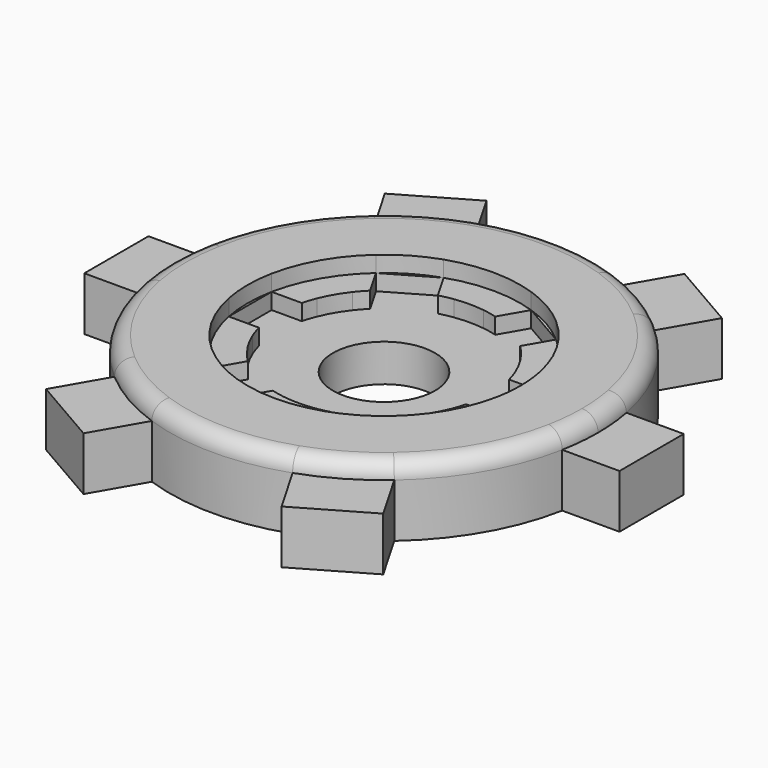
from build123d import *

# Parameters (mm, degrees)
F2_DEPTH = 2.54
F3_R     = 7.6884407039
F3_R_2   = 2.4226171542
F4_DEPTH = 1.778
F6_DEPTH = 0.762
F7_R     = 0.76199


# Not quite as in the source:
# - a fillet or chamfer is up to 0.001 mm smaller than in the source, because OpenCascade refuses the exact size


with BuildPart() as f2:
    # F1 (on Top) → F2 (new body)
    with BuildSketch(Plane.XY):
        with BuildLine():
            ThreePointArc((9.9798083649, -1.905), (10.1148517781, -0.9567515385), (10.16, 0))
            ThreePointArc((10.16, 0), (10.1148517781, 0.9567515385), (9.9798083649, 1.905))
            Line((9.9798083649, 1.905), (4.7092860393, 1.905))
            ThreePointArc((4.7092860393, 1.905), (4.8244462237, 1.5909489729), (4.9186888497, 1.27))
            Line((4.9186888497, 1.27), (6.35, 1.27))
            Line((6.35, 1.27), (6.35, -1.27))
            Line((6.35, -1.27), (4.9186888497, -1.27))
            ThreePointArc((4.9186888497, -1.27), (4.8244462237, -1.5909489729), (4.7092860393, -1.905))
            Line((4.7092860393, -1.905), (9.9798083649, -1.905))
        make_face()
        with BuildLine():
            ThreePointArc((9.9798083649, 1.905), (10.1148517781, 0.9567515385), (10.16, 0))
            ThreePointArc((10.16, 0), (10.1148517781, -0.9567515385), (9.9798083649, -1.905))
            Line((9.9798083649, -1.905), (12.7, -1.905))
            Line((12.7, -1.905), (12.7, 1.905))
            Line((12.7, 1.905), (9.9798083649, 1.905))
        make_face()
        with BuildLine():
            Line((4.7092860393, 1.905), (9.9798083649, 1.905))
            ThreePointArc((9.9798083649, 1.905), (8.7988181024, 5.08), (6.6396825767, 7.6902675689))
            Line((6.6396825767, 7.6902675689), (4.0044214139, 3.1258613437))
            ThreePointArc((4.0044214139, 3.1258613437), (4.3994090512, 2.54), (4.7092860393, 1.905))
        make_face()
        with BuildLine():
            ThreePointArc((6.6396825767, -7.6902675689), (8.7988181024, -5.08), (9.9798083649, -1.905))
            Line((9.9798083649, -1.905), (4.7092860393, -1.905))
            ThreePointArc((4.7092860393, -1.905), (4.3994090512, -2.54), (4.0044214139, -3.1258613437))
            Line((4.0044214139, -3.1258613437), (6.6396825767, -7.6902675689))
        make_face()
        with BuildLine():
            Line((4.0044214139, 3.1258613437), (6.6396825767, 7.6902675689))
            ThreePointArc((6.6396825767, 7.6902675689), (5.08, 8.7988181024), (3.3401257882, 9.5952675689))
            Line((3.3401257882, 9.5952675689), (0.7048646254, 5.0308613437))
            ThreePointArc((0.7048646254, 5.0308613437), (1.0344208852, 4.9735674754), (1.359492162, 4.8947094971))
            Line((1.359492162, 4.8947094971), (2.0751477372, 6.134261314))
            Line((2.0751477372, 6.134261314), (4.2748522628, 4.864261314))
            Line((4.2748522628, 4.864261314), (3.5591966876, 3.6247094971))
            ThreePointArc((3.5591966876, 3.6247094971), (3.7900253385, 3.3826185025), (4.0044214139, 3.1258613437))
        make_face()
        with BuildLine():
            ThreePointArc((3.3401257882, 9.5952675689), (5.08, 8.7988181024), (6.6396825767, 7.6902675689))
            Line((6.6396825767, 7.6902675689), (7.9997783942, 10.0460226281))
            Line((7.9997783942, 10.0460226281), (4.7002216058, 11.9510226281))
            Line((4.7002216058, 11.9510226281), (3.3401257882, 9.5952675689))
        make_face()
        with BuildLine():
            Line((7.9997783942, -10.0460226281), (6.6396825767, -7.6902675689))
            ThreePointArc((6.6396825767, -7.6902675689), (5.08, -8.7988181024), (3.3401257882, -9.5952675689))
            Line((3.3401257882, -9.5952675689), (4.7002216058, -11.9510226281))
            Line((4.7002216058, -11.9510226281), (7.9997783942, -10.0460226281))
        make_face()
        with BuildLine():
            ThreePointArc((3.3401257882, -9.5952675689), (5.08, -8.7988181024), (6.6396825767, -7.6902675689))
            Line((6.6396825767, -7.6902675689), (4.0044214139, -3.1258613437))
            ThreePointArc((4.0044214139, -3.1258613437), (3.7900253385, -3.3826185025), (3.5591966876, -3.6247094971))
            Line((3.5591966876, -3.6247094971), (4.2748522628, -4.864261314))
            Line((4.2748522628, -4.864261314), (2.0751477372, -6.134261314))
            Line((2.0751477372, -6.134261314), (1.359492162, -4.8947094971))
            ThreePointArc((1.359492162, -4.8947094971), (1.0344208852, -4.9735674754), (0.7048646254, -5.0308613437))
            Line((0.7048646254, -5.0308613437), (3.3401257882, -9.5952675689))
        make_face()
        with BuildLine():
            Line((0.7048646254, 5.0308613437), (3.3401257882, 9.5952675689))
            ThreePointArc((3.3401257882, 9.5952675689), (0, 10.16), (-3.3401257882, 9.5952675689))
            Line((-3.3401257882, 9.5952675689), (-0.7048646254, 5.0308613437))
            ThreePointArc((-0.7048646254, 5.0308613437), (0, 5.08), (0.7048646254, 5.0308613437))
        make_face()
        with BuildLine():
            ThreePointArc((-3.3401257882, -9.5952675689), (0, -10.16), (3.3401257882, -9.5952675689))
            Line((3.3401257882, -9.5952675689), (0.7048646254, -5.0308613437))
            ThreePointArc((0.7048646254, -5.0308613437), (0, -5.08), (-0.7048646254, -5.0308613437))
            Line((-0.7048646254, -5.0308613437), (-3.3401257882, -9.5952675689))
        make_face()
        with BuildLine():
            Line((-0.7048646254, 5.0308613437), (-3.3401257882, 9.5952675689))
            ThreePointArc((-3.3401257882, 9.5952675689), (-5.08, 8.7988181024), (-6.6396825767, 7.6902675689))
            Line((-6.6396825767, 7.6902675689), (-4.0044214139, 3.1258613437))
            ThreePointArc((-4.0044214139, 3.1258613437), (-3.7900253385, 3.3826185025), (-3.5591966876, 3.6247094971))
            Line((-3.5591966876, 3.6247094971), (-4.2748522628, 4.864261314))
            Line((-4.2748522628, 4.864261314), (-2.0751477372, 6.134261314))
            Line((-2.0751477372, 6.134261314), (-1.359492162, 4.8947094971))
            ThreePointArc((-1.359492162, 4.8947094971), (-1.0344208852, 4.9735674754), (-0.7048646254, 5.0308613437))
        make_face()
        with BuildLine():
            ThreePointArc((-6.6396825767, 7.6902675689), (-5.08, 8.7988181024), (-3.3401257882, 9.5952675689))
            Line((-3.3401257882, 9.5952675689), (-4.7002216058, 11.9510226281))
            Line((-4.7002216058, 11.9510226281), (-7.9997783942, 10.0460226281))
            Line((-7.9997783942, 10.0460226281), (-6.6396825767, 7.6902675689))
        make_face()
        with BuildLine():
            Line((-4.7002216058, -11.9510226281), (-3.3401257882, -9.5952675689))
            ThreePointArc((-3.3401257882, -9.5952675689), (-5.08, -8.7988181024), (-6.6396825767, -7.6902675689))
            Line((-6.6396825767, -7.6902675689), (-7.9997783942, -10.0460226281))
            Line((-7.9997783942, -10.0460226281), (-4.7002216058, -11.9510226281))
        make_face()
        with BuildLine():
            ThreePointArc((-6.6396825767, -7.6902675689), (-5.08, -8.7988181024), (-3.3401257882, -9.5952675689))
            Line((-3.3401257882, -9.5952675689), (-0.7048646254, -5.0308613437))
            ThreePointArc((-0.7048646254, -5.0308613437), (-1.0344208852, -4.9735674754), (-1.359492162, -4.8947094971))
            Line((-1.359492162, -4.8947094971), (-2.0751477372, -6.134261314))
            Line((-2.0751477372, -6.134261314), (-4.2748522628, -4.864261314))
            Line((-4.2748522628, -4.864261314), (-3.5591966876, -3.6247094971))
            ThreePointArc((-3.5591966876, -3.6247094971), (-3.7900253385, -3.3826185025), (-4.0044214139, -3.1258613437))
            Line((-4.0044214139, -3.1258613437), (-6.6396825767, -7.6902675689))
        make_face()
        with BuildLine():
            Line((-4.0044214139, 3.1258613437), (-6.6396825767, 7.6902675689))
            ThreePointArc((-6.6396825767, 7.6902675689), (-8.7988181024, 5.08), (-9.9798083649, 1.905))
            Line((-9.9798083649, 1.905), (-4.7092860393, 1.905))
            ThreePointArc((-4.7092860393, 1.905), (-4.3994090512, 2.54), (-4.0044214139, 3.1258613437))
        make_face()
        with BuildLine():
            ThreePointArc((-9.9798083649, -1.905), (-8.7988181024, -5.08), (-6.6396825767, -7.6902675689))
            Line((-6.6396825767, -7.6902675689), (-4.0044214139, -3.1258613437))
            ThreePointArc((-4.0044214139, -3.1258613437), (-4.3994090512, -2.54), (-4.7092860393, -1.905))
            Line((-4.7092860393, -1.905), (-9.9798083649, -1.905))
        make_face()
        with BuildLine():
            Line((-4.7092860393, 1.905), (-9.9798083649, 1.905))
            ThreePointArc((-9.9798083649, 1.905), (-10.16, 0), (-9.9798083649, -1.905))
            Line((-9.9798083649, -1.905), (-4.7092860393, -1.905))
            ThreePointArc((-4.7092860393, -1.905), (-4.8244462237, -1.5909489729), (-4.9186888497, -1.27))
            Line((-4.9186888497, -1.27), (-6.35, -1.27))
            Line((-6.35, -1.27), (-6.35, 1.27))
            Line((-6.35, 1.27), (-4.9186888497, 1.27))
            ThreePointArc((-4.9186888497, 1.27), (-4.8244462237, 1.5909489729), (-4.7092860393, 1.905))
        make_face()
        with BuildLine():
            ThreePointArc((-9.9798083649, -1.905), (-10.16, 0), (-9.9798083649, 1.905))
            Line((-9.9798083649, 1.905), (-12.7, 1.905))
            Line((-12.7, 1.905), (-12.7, -1.905))
            Line((-12.7, -1.905), (-9.9798083649, -1.905))
        make_face()
    extrude(amount=F2_DEPTH)

    # F3 (on face) → F4 (join)
    with BuildSketch(Plane.XY):
        Circle(F3_R)
        Circle(F3_R_2, mode=Mode.SUBTRACT)
    extrude(amount=F4_DEPTH)

    # F5 (on face) → F6 (join)
    with BuildSketch(Plane.XY.offset(2.54)):
        with BuildLine():
            ThreePointArc((9.9798083649, -1.905), (10.1148517781, -0.9567515385), (10.16, 0))
            ThreePointArc((10.16, 0), (10.1148517781, 0.9567515385), (9.9798083649, 1.905))
            ThreePointArc((9.9798083649, 1.905), (8.7988181024, 5.08), (6.6396825767, 7.6902675689))
            ThreePointArc((6.6396825767, 7.6902675689), (5.08, 8.7988181024), (3.3401257882, 9.5952675689))
            ThreePointArc((3.3401257882, 9.5952675689), (0, 10.16), (-3.3401257882, 9.5952675689))
            ThreePointArc((-3.3401257882, 9.5952675689), (-5.08, 8.7988181024), (-6.6396825767, 7.6902675689))
            ThreePointArc((-6.6396825767, 7.6902675689), (-8.7988181024, 5.08), (-9.9798083649, 1.905))
            ThreePointArc((-9.9798083649, 1.905), (-10.16, 0), (-9.9798083649, -1.905))
            ThreePointArc((-9.9798083649, -1.905), (-8.7988181024, -5.08), (-6.6396825767, -7.6902675689))
            ThreePointArc((-6.6396825767, -7.6902675689), (-5.08, -8.7988181024), (-3.3401257882, -9.5952675689))
            ThreePointArc((-3.3401257882, -9.5952675689), (0, -10.16), (3.3401257882, -9.5952675689))
            ThreePointArc((3.3401257882, -9.5952675689), (5.08, -8.7988181024), (6.6396825767, -7.6902675689))
            ThreePointArc((6.6396825767, -7.6902675689), (8.7988181024, -5.08), (9.9798083649, -1.905))
        make_face()
        with BuildLine():
            ThreePointArc((6.35, 1.27), (6.4442393992, 0.6381054508), (6.4757547823, 0))
            ThreePointArc((6.4757547823, 0), (6.4442393992, -0.6381054508), (6.35, -1.27))
            ThreePointArc((6.35, -1.27), (5.6081681501, -3.2378773911), (4.2748522628, -4.864261314))
            ThreePointArc((4.2748522628, -4.864261314), (3.2378773911, -5.6081681501), (2.0751477372, -6.134261314))
            ThreePointArc((2.0751477372, -6.134261314), (0, -6.4757547823), (-2.0751477372, -6.134261314))
            ThreePointArc((-2.0751477372, -6.134261314), (-3.2378773911, -5.6081681501), (-4.2748522628, -4.864261314))
            ThreePointArc((-4.2748522628, -4.864261314), (-5.6081681501, -3.2378773911), (-6.35, -1.27))
            ThreePointArc((-6.35, -1.27), (-6.4757547823, 0), (-6.35, 1.27))
            ThreePointArc((-6.35, 1.27), (-5.6081681501, 3.2378773911), (-4.2748522628, 4.864261314))
            ThreePointArc((-4.2748522628, 4.864261314), (-3.2378773911, 5.6081681501), (-2.0751477372, 6.134261314))
            ThreePointArc((-2.0751477372, 6.134261314), (0, 6.4757547823), (2.0751477372, 6.134261314))
            ThreePointArc((2.0751477372, 6.134261314), (3.2378773911, 5.6081681501), (4.2748522628, 4.864261314))
            ThreePointArc((4.2748522628, 4.864261314), (5.6081681501, 3.2378773911), (6.35, 1.27))
        make_face(mode=Mode.SUBTRACT)
    extrude(amount=F6_DEPTH)

    # F7 (radius 0.762 in the source; OpenCascade refuses exactly that, so slightly less here)
    f7_edges = [f2.edges().sort_by_distance(p)[0] for p in [
        (9.979808, 1.905, 3.302),
    ]]
    fillet(f7_edges, radius=F7_R)


solid = f2.part
